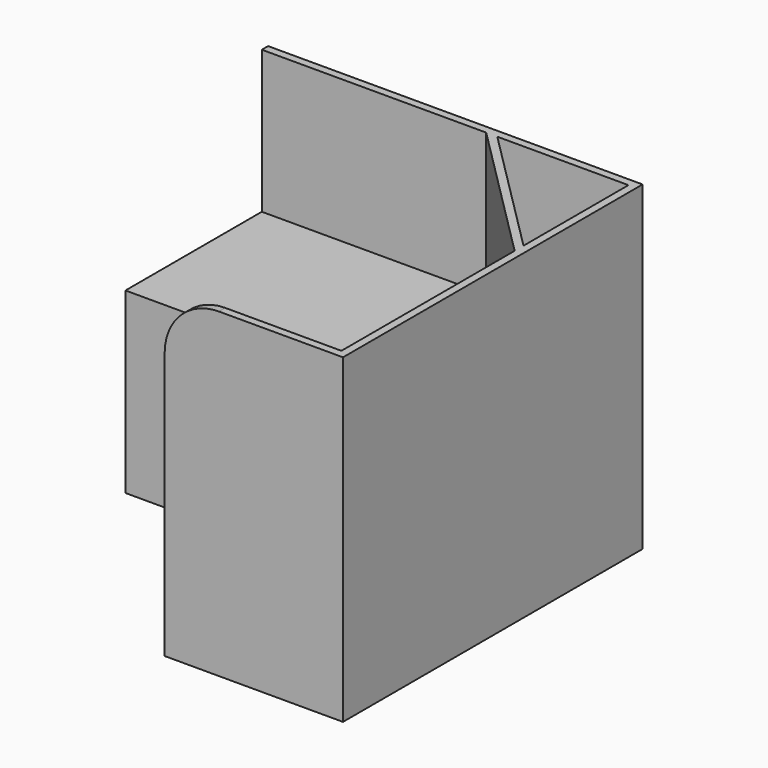
from build123d import *

# Parameters (mm, degrees)
F1_DEPTH = 500
F2_DEPTH = 400
F3_T     = -22
F5_DEPTH = 25


# Not quite as in the source:
# - a shell that OpenCascade refuses in one call is made with other operations: the cavity is built on its own and cut out


with BuildPart() as f1:
    # F0 (on Top) → F1 (new body)
    with BuildSketch(Plane.XY):
        Polygon((0, 0), (-1050, 0), (-1050, -22), (-420.8932188135, -22), (-22, -420.8932188135), (-22, -1028), (-500, -1028), (-500, -1050), (0, -1050), align=None)
        Polygon((-389.7805204412, -22), (-22, -22), (-22, -389.7805204412), align=None, mode=Mode.SUBTRACT)
        Polygon((-420.8932188135, -22), (-1050, -22), (-1050, -500), (-650, -500), (-500, -650), (-500, -1028), (-22, -1028), (-22, -420.8932188135), align=None)
    extrude(amount=-F1_DEPTH)

    # F0 (on Top) → F2 (join)
    with BuildSketch(Plane.XY):
        Polygon((0, 0), (-1050, 0), (-1050, -22), (-420.8932188135, -22), (-22, -420.8932188135), (-22, -1028), (-500, -1028), (-500, -1050), (0, -1050), align=None)
        Polygon((-389.7805204412, -22), (-22, -22), (-22, -389.7805204412), align=None, mode=Mode.SUBTRACT)
    extrude(amount=F2_DEPTH)

    # F3: a shell. OpenCascade refuses it in one call, so the cavity is built on its own and cut out:
    # the body offset inwards by the wall thickness, plus a prism from it out through each open face.
    f3_core = offset(f1.part, amount=F3_T, kind=Kind.INTERSECTION, mode=Mode.PRIVATE)
    f3_exits = [f3_core.faces().sort_by_distance(p)[0] for p in [
        (-463.695201, -463.695201, -478),
    ]]
    add(f3_core, mode=Mode.SUBTRACT)
    extrude(f3_exits, amount=-F3_T, mode=Mode.SUBTRACT)

    # F4 (on face) → F5 (cut)
    with BuildSketch(Plane.XZ.offset(1050)):
        with BuildLine():
            ThreePointArc((-500, 248), (-455.4802307404, 355.4802307404), (-348, 400))
            Line((-348, 400), (-500, 400))
            Line((-500, 400), (-500, 248))
        make_face()
    extrude(amount=-F5_DEPTH, mode=Mode.SUBTRACT)


solid = f1.part
